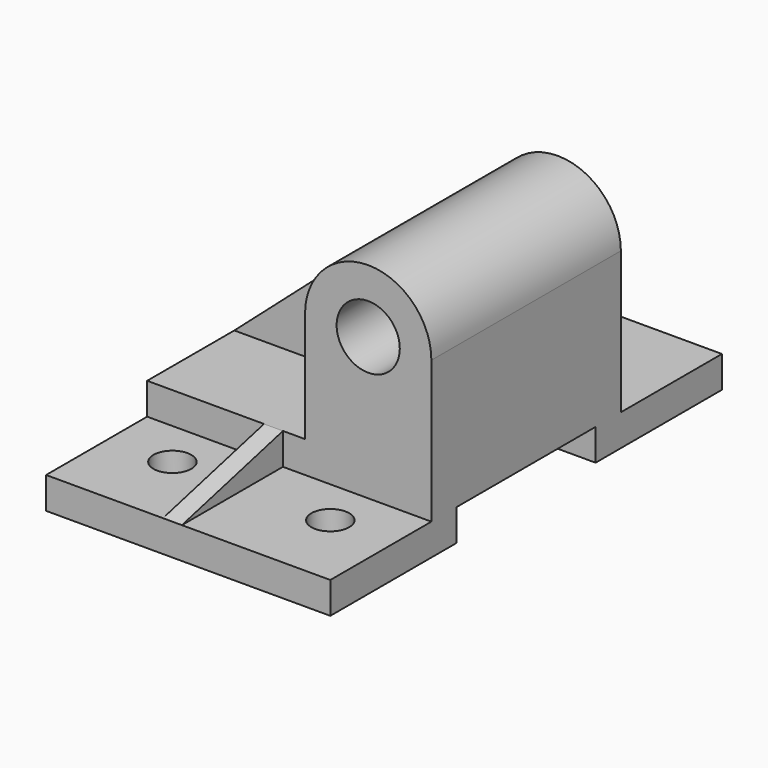
from build123d import *

# Parameters (mm, degrees)
F1_DEPTH  = 45
F2_R      = 6
F3_DEPTH  = 10.001
F6_DEPTH  = 6
F7_R      = 10
F8_DEPTH  = 37.5
F10_DEPTH = 3


# Not quite as in the source:
# - a pattern or mirror of a feature is missing from the dataset's text; its kind, count and spacing are read off the source's solid


with BuildPart() as f1:
    # F0 (on Right) → F1 (new body, symmetric)
    with BuildSketch(Plane.YZ):
        Polygon((27.5, -20), (77.5, -20), (77.5, -10), (37.5, -10), (37.5, 0), (-37.5, 0), (-37.5, -10), (-77.5, -10), (-77.5, -20), (-27.5, -20), (-27.5, -10), (27.5, -10), align=None)
    extrude(amount=F1_DEPTH, both=True)

    # F2 (on face) → F3 (cut, through all)
    with BuildSketch(Plane.XY.offset(-10)):
        with Locations((25, -52.5)):
            Circle(F2_R)
        with Locations((-25, -52.5)):
            Circle(F2_R)
        with Locations((-25, 52.5)):
            Circle(F2_R)
        with Locations((25, 52.5)):
            Circle(F2_R)
    extrude(amount=-F3_DEPTH, mode=Mode.SUBTRACT)

    # F5 (on offset) → F6 (join)
    with BuildSketch(Plane(origin=(-8, 0, 0), x_dir=(0, -1, 0), z_dir=(-1, 0, 0))):
        Polygon((-37.5, -10), (-37.5, 0), (-77.5, -10), align=None)
    f6 = extrude(amount=-F6_DEPTH)

    # F6_copies: F6 across plane
    add(f6.mirror(Plane(origin=(0, 0, 0), x_dir=(0, 0, -1), z_dir=(0, -1, 0))))

    # F7 (on Front) → F8 (join, symmetric)
    with BuildSketch(Plane.XZ):
        with BuildLine():
            Line((5, 0), (45, 0))
            Line((45, 0), (45, 35))
            ThreePointArc((45, 35), (25, 55), (5, 35))
            Line((5, 35), (5, 0))
        make_face()
        with Locations((25, 35)):
            Circle(F7_R, mode=Mode.SUBTRACT)
    extrude(amount=F8_DEPTH, both=True)

    # F9 (on Front) → F10 (join, symmetric)
    with BuildSketch(Plane.XZ):
        Polygon((11.7812880283, 50.0088525148), (-45, 0), (5, 0), align=None)
    extrude(amount=F10_DEPTH, both=True)


solid = f1.part
